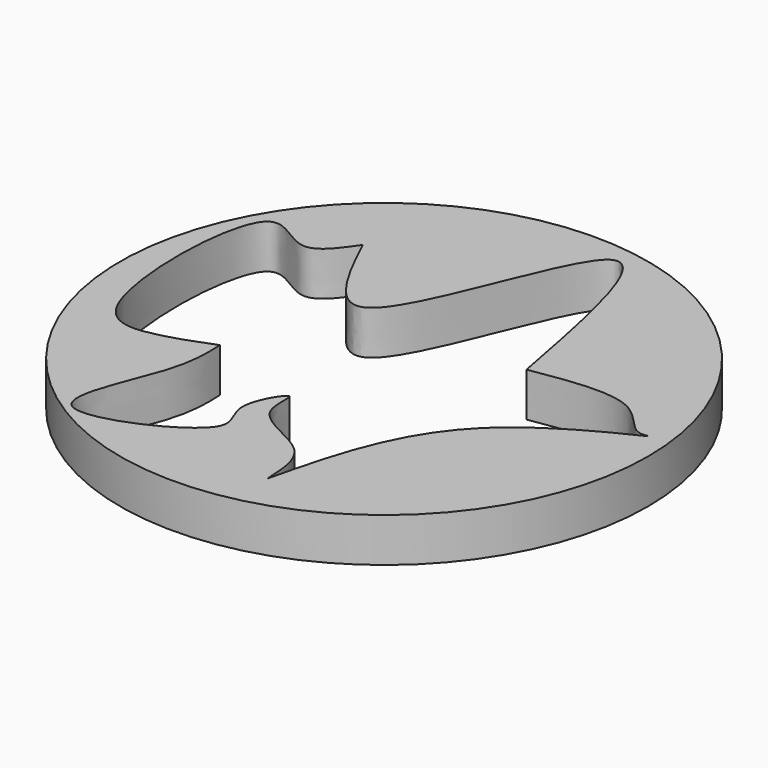
from build123d import *

# Parameters (mm, degrees)
F0_R     = 30
F1_DEPTH = 5


with BuildPart() as f1:
    # F0 (on Top) → F1 (new body)
    with BuildSketch(Plane.XY):
        Circle(F0_R)
        with BuildLine():
            add(Edge.make_bspline(
                [(11.1432595722, 6.3008036782), (15.5603060299, 7.0264709669), (22.9027823898, 8.2327509921), (25.8093539427, 2.5154011348), (29.6930561957, 3.8147112425), (11.2143468613, -3.8550044175), (8.0374621525, -17.0761381246), (6.2690470368, -24.4356915355)],
                knots=[0, 0, 0, 0, 0.2235288018, 0.3715729411, 0.4417269404, 0.6892369073, 1, 1, 1, 1], degree=3))
            add(Edge.make_bspline(
                [(6.2690470368, -24.4356915355), (6.1802657102, -22.1890257282), (5.9939706197, -17.4747144391), (-2.9736854852, -15.6823425273), (-1.1668697629, -8.6613601918), (-5.6221313444, -15.5957649297), (0.0286124979, -19.7014263791), (-21.1754449377, -29.3100378916), (-12.7765919914, -13.3349010401), (-12.9615218, -8.9747552381), (-13.0443992093, -7.0207295939)],
                knots=[0, 0, 0, 0, 0.1194409785, 0.2506300455, 0.3383614514, 0.4410934831, 0.5411512464, 0.7168949323, 0.8731247561, 1, 1, 1, 1], degree=3))
            add(Edge.make_bspline(
                [(-13.0443992093, -7.0207295939), (-14.9223158973, -7.761517675), (-18.6827252253, -9.2448989283), (-27.6128834737, -10.0300292339), (-27.1410394083, 19.7996455511), (-18.9645499436, 10.4482508336), (-16.4419179131, 14.1111670113), (-15.1802115142, 15.9431919456)],
                knots=[0, 0, 0, 0, 0.174575255, 0.3495759006, 0.6736770496, 0.8367880255, 1, 1, 1, 1], degree=3))
            add(Edge.make_bspline(
                [(-15.1802115142, 15.9431919456), (-12.5954163122, 10.5201087382), (-6.4167340587, -2.4432037696), (4.5506258251, 41.1929594406), (8.9613322001, 17.8488666607), (11.1432595722, 6.3008036782)],
                knots=[0, 0, 0, 0, 0.2665555825, 0.6371732066, 1, 1, 1, 1], degree=3))
        make_face(mode=Mode.SUBTRACT)
    extrude(amount=F1_DEPTH)


solid = f1.part
